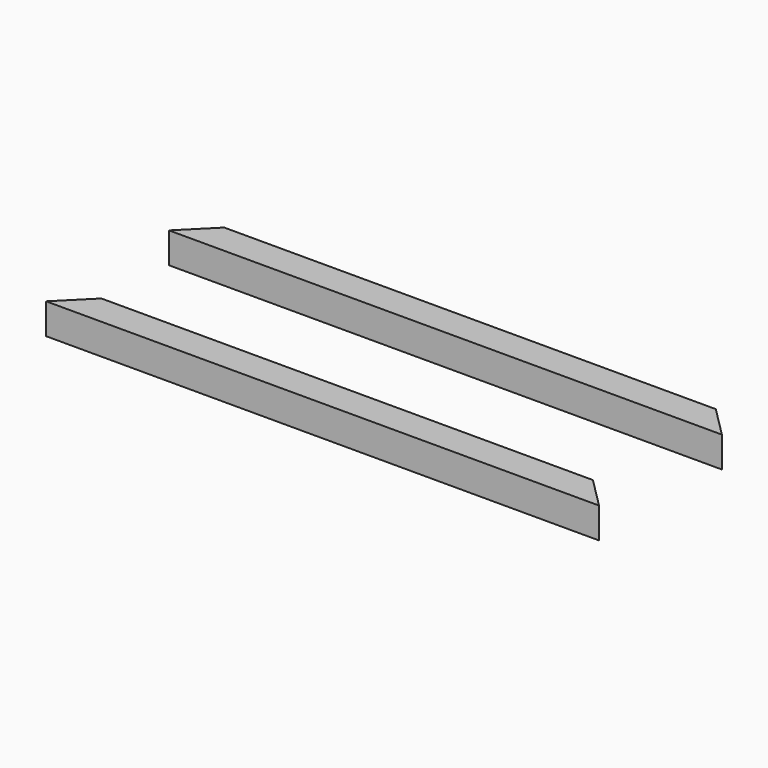
from build123d import *

# Parameters (mm, degrees)
F0_W        = 914.4
F0_H        = 50.8
F1_DEPTH    = 50.8
F2_W        = 44.45
F2_H        = 44.45
F3_DEPTH    = 914.401
F4_T1_DEPTH = 312.0829915773


# Not quite as in the source:
# - a fillet or chamfer that OpenCascade refuses, or shapes differently, is made with other operations: its cross-section is extruded or revolved along the edge and cut away or added


with BuildPart() as f1:
    # F0 (on Front) → F1 (new body)
    with BuildSketch(Plane.XZ):
        Rectangle(F0_W, F0_H)
    extrude(amount=F1_DEPTH)

    # F2 (on face) → F3 (cut, through all)
    with BuildSketch(Plane(origin=(-457.2, 0, 0), x_dir=(0, -1, 0), z_dir=(-1, 0, 0))):
        with Locations((25.4, 0)):
            Rectangle(F2_W, F2_H)
    extrude(amount=-F3_DEPTH, mode=Mode.SUBTRACT)

    # F4: chamfer of 50.8 on 2 edges, made by hand

    # F4_s2 → F4_t1 (cut)
    with BuildSketch(Plane.XY.offset(-156.0414957887)):
        Polygon((457.2, -50.8), (406.4, 0), (457.2, 0), align=None)
        Polygon((-406.4, 0), (-457.2, -50.8), (-457.2, 0), align=None)
    extrude(amount=F4_T1_DEPTH, mode=Mode.SUBTRACT)


with BuildPart() as f5_1:
    # F5: copy of F1
    add(f1.part.moved(Location((0, 254, 0))))


solid = Compound([f1.part, f5_1.part])
